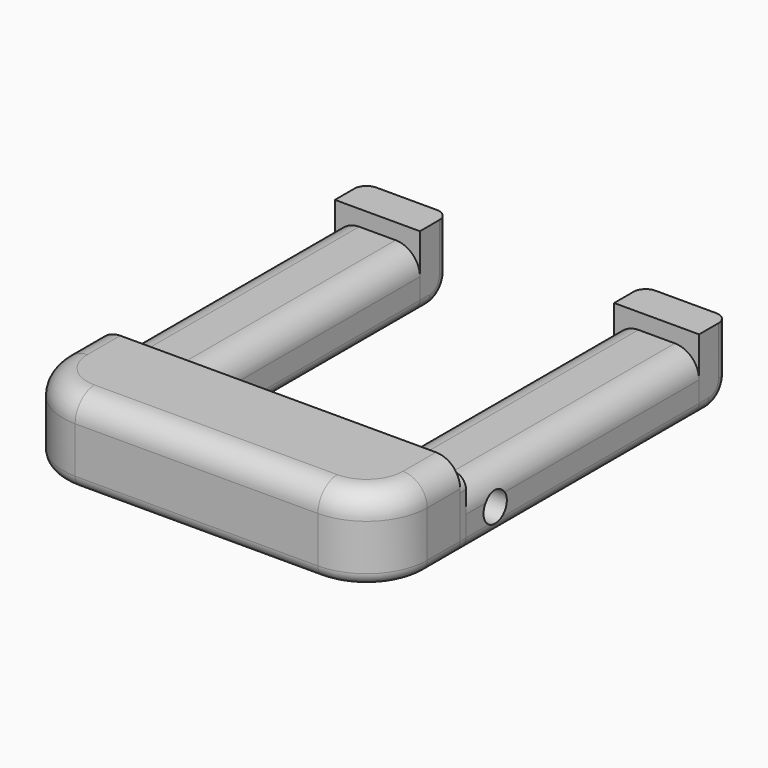
from build123d import *

# Parameters (mm, degrees)
F0_W         = 30
F0_H         = 8.4
F1_DEPTH     = 6.8
F0_W_2       = 7
F0_H_2       = 24
F2_DEPTH     = 4.7
F0_H_3       = 3
F3_DEPTH     = 6
F4_DEPTH     = 5.5
F5_R         = 2
F5_2_R       = 2
F5_3_R       = 2
F5_4_R       = 2
F5_5_R       = 2
F6_R         = 1
F7_R         = 1
F7_2_R       = 1
F7_3_R       = 1
F7_4_R       = 1
F7_5_R       = 1
F7_6_R       = 1
F8_T1_DEPTH  = 6.8
F8_T4_ANGLE  = 90
F8_T6_ANGLE  = 90
F8_T8_ANGLE  = 90
F8_T10_ANGLE = 90
F9_R         = 1.2
F10_DEPTH    = 55.5


# Not quite as in the source:
# - a fillet or chamfer that OpenCascade refuses, or shapes differently, is made with other operations: its cross-section is extruded or revolved along the edge and cut away or added


with BuildPart() as f1:
    # F0 (on Top) → F1 (new body)
    with BuildSketch(Plane.XY):
        with Locations((0, 4.2)):
            Rectangle(F0_W, F0_H)
    extrude(amount=F1_DEPTH)

    # F5#3
    f5_3_edges = [f1.edges().sort_by_distance(p)[0] for p in [
        (15, 4.2, 6.8),
        (-15, 4.2, 6.8),
        (0, 0, 6.8),
    ]]
    fillet(f5_3_edges, radius=F5_3_R)

    # F7#4
    f7_4_edges = [f1.edges().sort_by_distance(p)[0] for p in [
        (15, 4.2, 0),
        (0, 0, 0),
        (-15, 4.2, 0),
    ]]
    fillet(f7_4_edges, radius=F7_4_R)

    # F8: fillet of radius 5 on 2 edges, made by hand

    # F8_s2 → F8_t1 (cut)
    with BuildSketch(Plane.XY):
        with BuildLine():
            ThreePointArc((15, 5), (13.5355339059, 1.4644660941), (10, 0))
            Line((10, 0), (15, 0))
            Line((15, 0), (15, 5))
        make_face()
        with BuildLine():
            ThreePointArc((-15, 5), (-13.5355339059, 1.4644660941), (-10, 0))
            Line((-10, 0), (-15, 0))
            Line((-15, 0), (-15, 5))
        make_face()
    extrude(amount=F8_T1_DEPTH, mode=Mode.SUBTRACT)

    # F8_s3 → F8_t4 (revolve, cut)
    with BuildSketch(Plane.YZ.offset(-10)):
        with BuildLine():
            ThreePointArc((1, 0), (0.2928932188, 0.2928932188), (0, 1))
            Line((0, 1), (0, 0))
            Line((0, 0), (1, 0))
        make_face()
    revolve(axis=Axis((-10, 5, 0), (0, 0, -1)), revolution_arc=F8_T4_ANGLE, mode=Mode.SUBTRACT)

    # F8_s5 → F8_t6 (revolve, cut)
    with BuildSketch(Plane.XZ.offset(-5)):
        with BuildLine():
            ThreePointArc((-13, 6.8), (-14.4142135624, 6.2142135624), (-15, 4.8))
            Line((-15, 4.8), (-15, 6.8))
            Line((-15, 6.8), (-13, 6.8))
        make_face()
    revolve(axis=Axis((-10, 5, 6.8), (0, 0, 1)), revolution_arc=F8_T6_ANGLE, mode=Mode.SUBTRACT)

    # F8_s7 → F8_t8 (revolve, cut)
    with BuildSketch(Plane.XZ.offset(-5)):
        with BuildLine():
            ThreePointArc((14, 0), (14.7071067812, 0.2928932188), (15, 1))
            Line((15, 1), (15, 0))
            Line((15, 0), (14, 0))
        make_face()
    revolve(axis=Axis((10, 5, 0), (0, 0, -1)), revolution_arc=F8_T8_ANGLE, mode=Mode.SUBTRACT)

    # F8_s9 → F8_t10 (revolve, cut)
    with BuildSketch(Plane.YZ.offset(10)):
        with BuildLine():
            ThreePointArc((2, 6.8), (0.5857864376, 6.2142135624), (0, 4.8))
            Line((0, 4.8), (0, 6.8))
            Line((0, 6.8), (2, 6.8))
        make_face()
    revolve(axis=Axis((10, 5, 6.8), (0, 0, 1)), revolution_arc=F8_T10_ANGLE, mode=Mode.SUBTRACT)


with BuildPart() as f2:
    # F0 (on Top) → F2 (new body)
    with BuildSketch(Plane.XY):
        with Locations((-11.5, 21)):
            Rectangle(F0_W_2, F0_H_2)
    extrude(amount=F2_DEPTH)

    # F5#4
    f5_4_edges = [f2.edges().sort_by_distance(p)[0] for p in [
        (-15, 21, 4.7),
        (-8, 21, 4.7),
    ]]
    fillet(f5_4_edges, radius=F5_4_R)

    # F7#5
    f7_5_edges = [f2.edges().sort_by_distance(p)[0] for p in [
        (-8, 21, 0),
        (-15, 21, 0),
    ]]
    fillet(f7_5_edges, radius=F7_5_R)


with BuildPart() as f2b:
    # F0 (on Top) → F2, piece 2 (new body)
    with BuildSketch(Plane.XY):
        with Locations((11.5, 21)):
            Rectangle(F0_W_2, F0_H_2)
    extrude(amount=F2_DEPTH)

    # F5#5
    f5_5_edges = [f2b.edges().sort_by_distance(p)[0] for p in [
        (8, 21, 4.7),
        (15, 21, 4.7),
    ]]
    fillet(f5_5_edges, radius=F5_5_R)

    # F7#2
    f7_2_edges = [f2b.edges().sort_by_distance(p)[0] for p in [
        (15, 21, 0),
        (8, 21, 0),
    ]]
    fillet(f7_2_edges, radius=F7_2_R)


with BuildPart() as f3:
    # F0 (on Top) → F3 (new body)
    with BuildSketch(Plane.XY):
        with Locations((-11.5, 34.5)):
            Rectangle(F0_W_2, F0_H_3)
    extrude(amount=F3_DEPTH)

    # F5#2
    f5_2_edges = [f3.edges().sort_by_distance(p)[0] for p in [
        (-11.5, 36, 0),
    ]]
    fillet(f5_2_edges, radius=F5_2_R)

    # F7#6
    f7_6_edges = [f3.edges().sort_by_distance(p)[0] for p in [
        (-15, 33.5, 0),
        (-15, 35.414214, 0.585786),
        (-8, 33.5, 0),
        (-8, 35.414214, 0.585786),
        (-15, 36, 4),
        (-8, 36, 4),
    ]]
    fillet(f7_6_edges, radius=F7_6_R)


with BuildPart() as f3b:
    # F0 (on Top) → F3, piece 2 (new body)
    with BuildSketch(Plane.XY):
        with Locations((11.5, 34.5)):
            Rectangle(F0_W_2, F0_H_3)
    extrude(amount=F3_DEPTH)

    # F5
    f5_edges = [f3b.edges().sort_by_distance(p)[0] for p in [
        (11.5, 36, 0),
    ]]
    fillet(f5_edges, radius=F5_R)

    # F7
    f7_edges = [f3b.edges().sort_by_distance(p)[0] for p in [
        (15, 33.5, 0),
        (15, 35.414214, 0.585786),
        (8, 33.5, 0),
        (8, 35.414214, 0.585786),
        (8, 36, 4),
        (15, 36, 4),
    ]]
    fillet(f7_edges, radius=F7_R)


with BuildPart() as f4:
    # F0 (on Top) → F4 (new body)
    with BuildSketch(Plane.XY):
        Polygon((-8, 9), (-15, 9), (-15, 8.4), (15, 8.4), (15, 9), (8, 9), align=None)
    extrude(amount=F4_DEPTH)

    # F6
    f6_edges = [f4.edges().sort_by_distance(p)[0] for p in [
        (15, 8.7, 5.5),
        (-15, 8.7, 5.5),
    ]]
    fillet(f6_edges, radius=F6_R)

    # F7#3
    f7_3_edges = [f4.edges().sort_by_distance(p)[0] for p in [
        (15, 8.7, 0),
        (-15, 8.7, 0),
    ]]
    fillet(f7_3_edges, radius=F7_3_R)


with BuildPart() as f10_tool:
    # F9 (on Right) → F10 (new body, symmetric)
    with BuildSketch(Plane.YZ):
        with Locations((12, 2.0145524759)):
            Circle(F9_R)
    extrude(amount=F10_DEPTH, both=True)


with BuildPart() as f2_1:
    add(f2.part)

    # F10: cut by f10_tool
    add(f10_tool.part, mode=Mode.SUBTRACT)


with BuildPart() as f2b_1:
    add(f2b.part)

    # F10: cut by f10_tool
    add(f10_tool.part, mode=Mode.SUBTRACT)


solid = Compound([f1.part, f3.part, f3b.part, f4.part, f2_1.part, f2b_1.part])
